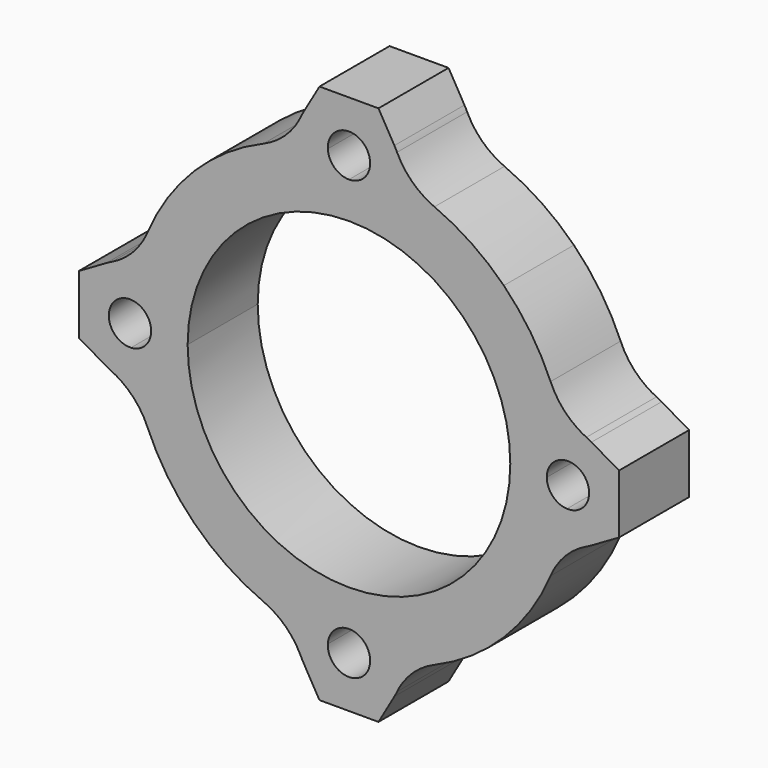
from build123d import *

# Parameters (mm, degrees)
F1_DEPTH     = 6
F2_T1_DEPTH  = 15.3027934974
F3_R         = 5
F4_T1_DEPTH  = 15.3027934974
F5_R         = 5
F6_T1_DEPTH  = 15.3027934974
F7_R         = 5
F8_T1_DEPTH  = 15.3027934974
F9_R         = 5
F10_T1_DEPTH = 15.3027934974
F11_R        = 5
F12_T1_DEPTH = 15.3027934974
F13_R        = 5
F14_R        = 2.75
F15_DEPTH    = 2.9


# Not quite as in the source:
# - a fillet or chamfer that OpenCascade refuses, or shapes differently, is made with other operations: its cross-section is extruded or revolved along the edge and cut away or added


with BuildPart() as f1:
    # F0 (on Front) → F1 (new body)
    with BuildSketch(Plane.XZ):
        with BuildLine():
            Line((11.5, 0), (11.05, 0))
            ThreePointArc((11.05, 0), (0, -11.05), (-11.05, 0))
            Line((-11.05, 0), (-11.5, 0))
            Line((-11.5, 0), (-11.5, -2.0207259422))
            Line((-11.5, -2.0207259422), (-14.5199840255, -3.7643145323))
            ThreePointArc((-14.5199840255, -3.7643145323), (-10.6066017178, -10.6066017178), (-3.7643145323, -14.5199840255))
            Line((-3.7643145323, -14.5199840255), (-2.0207259422, -11.5))
            Line((-2.0207259422, -11.5), (2.0207259422, -11.5))
            Line((2.0207259422, -11.5), (3.7643145323, -14.5199840255))
            ThreePointArc((3.7643145323, -14.5199840255), (10.6066017178, -10.6066017178), (14.5199840255, -3.7643145323))
            Line((14.5199840255, -3.7643145323), (11.5, -2.0207259422))
            Line((11.5, -2.0207259422), (11.5, 0))
        make_face()
        with BuildLine():
            ThreePointArc((7.8135299321, 7.8135299321), (10.2088688342, 4.2286519276), (11.05, 0))
            Line((11.05, 0), (11.5, 0))
            Line((11.5, 0), (11.5, 2.0207259422))
            Line((11.5, 2.0207259422), (14.5199840255, 3.7643145323))
            ThreePointArc((14.5199840255, 3.7643145323), (13.020773835, 7.4471100931), (10.6066017178, 10.6066017178))
            Line((10.6066017178, 10.6066017178), (7.8135299321, 7.8135299321))
        make_face()
        with BuildLine():
            ThreePointArc((0, 11.05), (4.2286519276, 10.2088688342), (7.8135299321, 7.8135299321))
            Line((7.8135299321, 7.8135299321), (10.6066017178, 10.6066017178))
            ThreePointArc((10.6066017178, 10.6066017178), (7.4471100931, 13.020773835), (3.7643145323, 14.5199840255))
            Line((3.7643145323, 14.5199840255), (2.0207259422, 11.5))
            Line((2.0207259422, 11.5), (0, 11.5))
            Line((0, 11.5), (0, 11.05))
        make_face()
        with BuildLine():
            Line((-11.5, 0), (-11.05, 0))
            ThreePointArc((-11.05, 0), (-7.8135299321, 7.8135299321), (0, 11.05))
            Line((0, 11.05), (0, 11.5))
            Line((0, 11.5), (-2.0207259422, 11.5))
            Line((-2.0207259422, 11.5), (-3.7643145323, 14.5199840255))
            ThreePointArc((-3.7643145323, 14.5199840255), (-10.6066017178, 10.6066017178), (-14.5199840255, 3.7643145323))
            Line((-14.5199840255, 3.7643145323), (-11.5, 2.0207259422))
            Line((-11.5, 2.0207259422), (-11.5, 0))
        make_face()
        with BuildLine():
            Line((11.5, 2.0207259422), (11.5, 0))
            Line((11.5, 0), (13.55, 0))
            ThreePointArc((13.55, 0), (13.9502093463, 1.0002197675), (14.9299166667, 1.4483053291))
            ThreePointArc((14.9299166667, 1.4483053291), (14.770414258, 2.6143570237), (14.5199840255, 3.7643145323))
            Line((14.5199840255, 3.7643145323), (11.5, 2.0207259422))
        make_face()
        with BuildLine():
            Line((13.55, 0), (11.5, 0))
            Line((11.5, 0), (11.5, -2.0207259422))
            Line((11.5, -2.0207259422), (14.5199840255, -3.7643145323))
            ThreePointArc((14.5199840255, -3.7643145323), (14.770414258, -2.6143570237), (14.9299166667, -1.4483053291))
            ThreePointArc((14.9299166667, -1.4483053291), (13.9502093463, -1.0002197675), (13.55, 0))
        make_face()
        with BuildLine():
            Line((-11.5, -2.0207259422), (-11.5, 0))
            Line((-11.5, 0), (-13.55, 0))
            ThreePointArc((-13.55, 0), (-13.9502093463, -1.0002197675), (-14.9299166667, -1.4483053291))
            ThreePointArc((-14.9299166667, -1.4483053291), (-14.770414258, -2.6143570237), (-14.5199840255, -3.7643145323))
            Line((-14.5199840255, -3.7643145323), (-11.5, -2.0207259422))
        make_face()
        with BuildLine():
            Line((-13.55, 0), (-11.5, 0))
            Line((-11.5, 0), (-11.5, 2.0207259422))
            Line((-11.5, 2.0207259422), (-14.5199840255, 3.7643145323))
            ThreePointArc((-14.5199840255, 3.7643145323), (-14.770414258, 2.6143570237), (-14.9299166667, 1.4483053291))
            ThreePointArc((-14.9299166667, 1.4483053291), (-13.9502093463, 1.0002197675), (-13.55, 0))
        make_face()
        with BuildLine():
            Line((0, 13.55), (0, 11.5))
            Line((0, 11.5), (2.0207259422, 11.5))
            Line((2.0207259422, 11.5), (3.7643145323, 14.5199840255))
            ThreePointArc((3.7643145323, 14.5199840255), (2.6143570237, 14.770414258), (1.4483053291, 14.9299166667))
            ThreePointArc((1.4483053291, 14.9299166667), (1.0002197675, 13.9502093463), (0, 13.55))
        make_face()
        with BuildLine():
            Line((-2.0207259422, 11.5), (0, 11.5))
            Line((0, 11.5), (0, 13.55))
            ThreePointArc((0, 13.55), (-1.0002197675, 13.9502093463), (-1.4483053291, 14.9299166667))
            ThreePointArc((-1.4483053291, 14.9299166667), (-2.6143570237, 14.770414258), (-3.7643145323, 14.5199840255))
            Line((-3.7643145323, 14.5199840255), (-2.0207259422, 11.5))
        make_face()
        with BuildLine():
            Line((15, 4.0414518843), (14.5199840255, 3.7643145323))
            ThreePointArc((14.5199840255, 3.7643145323), (14.770414258, 2.6143570237), (14.9299166667, 1.4483053291))
            ThreePointArc((14.9299166667, 1.4483053291), (16.0002197675, 1.0497906537), (16.45, 0))
            ThreePointArc((16.45, 0), (16.0002197675, -1.0497906537), (14.9299166667, -1.4483053291))
            ThreePointArc((14.9299166667, -1.4483053291), (14.770414258, -2.6143570237), (14.5199840255, -3.7643145323))
            Line((14.5199840255, -3.7643145323), (15, -4.0414518843))
            Line((15, -4.0414518843), (18.5, -2.0207259422))
            Line((18.5, -2.0207259422), (18.5, 2.0207259422))
            Line((18.5, 2.0207259422), (15, 4.0414518843))
        make_face()
        with BuildLine():
            ThreePointArc((1.4483053291, 14.9299166667), (2.6143570237, 14.770414258), (3.7643145323, 14.5199840255))
            Line((3.7643145323, 14.5199840255), (4.0414518843, 15))
            Line((4.0414518843, 15), (2.0207259422, 18.5))
            Line((2.0207259422, 18.5), (-2.0207259422, 18.5))
            Line((-2.0207259422, 18.5), (-4.0414518843, 15))
            Line((-4.0414518843, 15), (-3.7643145323, 14.5199840255))
            ThreePointArc((-3.7643145323, 14.5199840255), (-2.6143570237, 14.770414258), (-1.4483053291, 14.9299166667))
            ThreePointArc((-1.4483053291, 14.9299166667), (-0.0350519098, 16.4495762704), (1.45, 15))
            ThreePointArc((1.45, 15), (1.4495762704, 14.9649480902), (1.4483053291, 14.9299166667))
        make_face()
        with BuildLine():
            ThreePointArc((-14.9299166667, -1.4483053291), (-16.45, 0), (-14.9299166667, 1.4483053291))
            ThreePointArc((-14.9299166667, 1.4483053291), (-14.770414258, 2.6143570237), (-14.5199840255, 3.7643145323))
            Line((-14.5199840255, 3.7643145323), (-15, 4.0414518843))
            Line((-15, 4.0414518843), (-18.5, 2.0207259422))
            Line((-18.5, 2.0207259422), (-18.5, -2.0207259422))
            Line((-18.5, -2.0207259422), (-15, -4.0414518843))
            Line((-15, -4.0414518843), (-14.5199840255, -3.7643145323))
            ThreePointArc((-14.5199840255, -3.7643145323), (-14.770414258, -2.6143570237), (-14.9299166667, -1.4483053291))
        make_face()
        with BuildLine():
            Line((4.0414518843, -15), (3.7643145323, -14.5199840255))
            ThreePointArc((3.7643145323, -14.5199840255), (2.6143570237, -14.770414258), (1.4483053291, -14.9299166667))
            ThreePointArc((1.4483053291, -14.9299166667), (1.4495762704, -14.9649480902), (1.45, -15))
            ThreePointArc((1.45, -15), (-0.0350519098, -16.4495762704), (-1.4483053291, -14.9299166667))
            ThreePointArc((-1.4483053291, -14.9299166667), (-2.6143570237, -14.770414258), (-3.7643145323, -14.5199840255))
            Line((-3.7643145323, -14.5199840255), (-4.0414518843, -15))
            Line((-4.0414518843, -15), (-2.0207259422, -18.5))
            Line((-2.0207259422, -18.5), (2.0207259422, -18.5))
            Line((2.0207259422, -18.5), (4.0414518843, -15))
        make_face()
        with BuildLine():
            ThreePointArc((1.4483053291, -14.9299166667), (2.6143570237, -14.770414258), (3.7643145323, -14.5199840255))
            Line((3.7643145323, -14.5199840255), (2.0207259422, -11.5))
            Line((2.0207259422, -11.5), (-2.0207259422, -11.5))
            Line((-2.0207259422, -11.5), (-3.7643145323, -14.5199840255))
            ThreePointArc((-3.7643145323, -14.5199840255), (-2.6143570237, -14.770414258), (-1.4483053291, -14.9299166667))
            ThreePointArc((-1.4483053291, -14.9299166667), (0, -13.55), (1.4483053291, -14.9299166667))
        make_face()
    extrude(amount=F1_DEPTH)

    # F2: fillet of radius 5 on 1 edges, made by hand

    # F2_s2 → F2_t1 (cut)
    with BuildSketch(Plane.XZ.offset(-4.6513967487)):
        with BuildLine():
            ThreePointArc((-3.1111725346, 16.611291099), (-3.5536996774, 15.6018521519), (-3.7643145323, 14.5199840255))
            Line((-3.7643145323, 14.5199840255), (-3.8639799126, 14.5281578841))
            ThreePointArc((-3.8639799126, 14.5281578841), (-3.9894857487, 14.7099920128), (-4.1280544247, 14.95))
            Line((-4.1280544247, 14.95), (-4.1280544247, 15.05))
            Line((-4.1280544247, 15.05), (-3.197775075, 16.661291099))
            Line((-3.197775075, 16.661291099), (-3.1111725346, 16.611291099))
        make_face()
    extrude(amount=F2_T1_DEPTH, mode=Mode.SUBTRACT)

    # F3
    f3_edges = [f1.edges().sort_by_distance(p)[0] for p in [
        (-3.764315, -3, 14.519984),
    ]]
    fillet(f3_edges, radius=F3_R)

    # F4: fillet of radius 5 on 1 edges, made by hand

    # F4_s2 → F4_t1 (cut)
    with BuildSketch(Plane.XZ.offset(-4.6513967487)):
        with BuildLine():
            ThreePointArc((3.1111725346, 16.611291099), (3.5536996774, 15.6018521519), (3.7643145323, 14.5199840255))
            Line((3.7643145323, 14.5199840255), (3.8639799126, 14.5281578841))
            ThreePointArc((3.8639799126, 14.5281578841), (3.9894857487, 14.7099920128), (4.1280544247, 14.95))
            Line((4.1280544247, 14.95), (4.1280544247, 15.05))
            Line((4.1280544247, 15.05), (3.197775075, 16.661291099))
            Line((3.197775075, 16.661291099), (3.1111725346, 16.611291099))
        make_face()
    extrude(amount=F4_T1_DEPTH, mode=Mode.SUBTRACT)

    # F5
    f5_edges = [f1.edges().sort_by_distance(p)[0] for p in [
        (3.764315, -3, 14.519984),
    ]]
    fillet(f5_edges, radius=F5_R)

    # F6: fillet of radius 5 on 2 edges, made by hand

    # F6_s2 → F6_t1 (cut)
    with BuildSketch(Plane.XZ.offset(-4.6513967487)):
        with BuildLine():
            ThreePointArc((14.5199840255, 3.7643145323), (15.6018521519, 3.5536996774), (16.611291099, 3.1111725346))
            Line((16.611291099, 3.1111725346), (16.661291099, 3.197775075))
            Line((16.661291099, 3.197775075), (15.05, 4.1280544247))
            Line((15.05, 4.1280544247), (14.95, 4.1280544247))
            ThreePointArc((14.95, 4.1280544247), (14.7099920128, 3.9894857487), (14.5281578841, 3.8639799126))
            Line((14.5281578841, 3.8639799126), (14.5199840255, 3.7643145323))
        make_face()
        with BuildLine():
            ThreePointArc((16.611291099, -3.1111725346), (15.6018521519, -3.5536996774), (14.5199840255, -3.7643145323))
            Line((14.5199840255, -3.7643145323), (14.5281578841, -3.8639799126))
            ThreePointArc((14.5281578841, -3.8639799126), (14.7099920128, -3.9894857487), (14.95, -4.1280544247))
            Line((14.95, -4.1280544247), (15.05, -4.1280544247))
            Line((15.05, -4.1280544247), (16.661291099, -3.197775075))
            Line((16.661291099, -3.197775075), (16.611291099, -3.1111725346))
        make_face()
    extrude(amount=F6_T1_DEPTH, mode=Mode.SUBTRACT)

    # F7
    f7_edges = [f1.edges().sort_by_distance(p)[0] for p in [
        (14.519984, -3, 3.764315),
        (14.519984, -3, -3.764315),
    ]]
    fillet(f7_edges, radius=F7_R)

    # F8: fillet of radius 5 on 1 edges, made by hand

    # F8_s2 → F8_t1 (cut)
    with BuildSketch(Plane.XZ.offset(-4.6513967487)):
        with BuildLine():
            ThreePointArc((-3.1111725346, -16.611291099), (-3.5536996774, -15.6018521519), (-3.7643145323, -14.5199840255))
            Line((-3.7643145323, -14.5199840255), (-3.8639799126, -14.5281578841))
            ThreePointArc((-3.8639799126, -14.5281578841), (-3.9894857487, -14.7099920128), (-4.1280544247, -14.95))
            Line((-4.1280544247, -14.95), (-4.1280544247, -15.05))
            Line((-4.1280544247, -15.05), (-3.197775075, -16.661291099))
            Line((-3.197775075, -16.661291099), (-3.1111725346, -16.611291099))
        make_face()
    extrude(amount=F8_T1_DEPTH, mode=Mode.SUBTRACT)

    # F9
    f9_edges = [f1.edges().sort_by_distance(p)[0] for p in [
        (-3.764315, -3, -14.519984),
    ]]
    fillet(f9_edges, radius=F9_R)

    # F10: fillet of radius 5 on 1 edges, made by hand

    # F10_s2 → F10_t1 (cut)
    with BuildSketch(Plane.XZ.offset(-4.6513967487)):
        with BuildLine():
            ThreePointArc((3.1111725346, -16.611291099), (3.5536996774, -15.6018521519), (3.7643145323, -14.5199840255))
            Line((3.7643145323, -14.5199840255), (3.8639799126, -14.5281578841))
            ThreePointArc((3.8639799126, -14.5281578841), (3.9894857487, -14.7099920128), (4.1280544247, -14.95))
            Line((4.1280544247, -14.95), (4.1280544247, -15.05))
            Line((4.1280544247, -15.05), (3.197775075, -16.661291099))
            Line((3.197775075, -16.661291099), (3.1111725346, -16.611291099))
        make_face()
    extrude(amount=F10_T1_DEPTH, mode=Mode.SUBTRACT)

    # F11
    f11_edges = [f1.edges().sort_by_distance(p)[0] for p in [
        (3.764315, -3, -14.519984),
    ]]
    fillet(f11_edges, radius=F11_R)

    # F12: fillet of radius 5 on 2 edges, made by hand

    # F12_s2 → F12_t1 (cut)
    with BuildSketch(Plane.XZ.offset(-4.6513967487)):
        with BuildLine():
            ThreePointArc((-14.5199840255, -3.7643145323), (-15.6018521519, -3.5536996774), (-16.611291099, -3.1111725346))
            Line((-16.611291099, -3.1111725346), (-16.661291099, -3.197775075))
            Line((-16.661291099, -3.197775075), (-15.05, -4.1280544247))
            Line((-15.05, -4.1280544247), (-14.95, -4.1280544247))
            ThreePointArc((-14.95, -4.1280544247), (-14.7099920128, -3.9894857487), (-14.5281578841, -3.8639799126))
            Line((-14.5281578841, -3.8639799126), (-14.5199840255, -3.7643145323))
        make_face()
        with BuildLine():
            ThreePointArc((-16.611291099, 3.1111725346), (-15.6018521519, 3.5536996774), (-14.5199840255, 3.7643145323))
            Line((-14.5199840255, 3.7643145323), (-14.5281578841, 3.8639799126))
            ThreePointArc((-14.5281578841, 3.8639799126), (-14.7099920128, 3.9894857487), (-14.95, 4.1280544247))
            Line((-14.95, 4.1280544247), (-15.05, 4.1280544247))
            Line((-15.05, 4.1280544247), (-16.661291099, 3.197775075))
            Line((-16.661291099, 3.197775075), (-16.611291099, 3.1111725346))
        make_face()
    extrude(amount=F12_T1_DEPTH, mode=Mode.SUBTRACT)

    # F13
    f13_edges = [f1.edges().sort_by_distance(p)[0] for p in [
        (-14.519984, -3, 3.764315),
        (-14.519984, -3, -3.764315),
    ]]
    fillet(f13_edges, radius=F13_R)

    # F14 (on Front) → F15 (cut)
    with BuildSketch(Plane.XZ):
        with Locations((0, 15)):
            Circle(F14_R)
        with Locations((0, -15)):
            Circle(F14_R)
        with Locations((15, 0)):
            Circle(F14_R)
        with Locations((-15, 0)):
            Circle(F14_R)
    extrude(amount=F15_DEPTH, mode=Mode.SUBTRACT)


solid = f1.part
